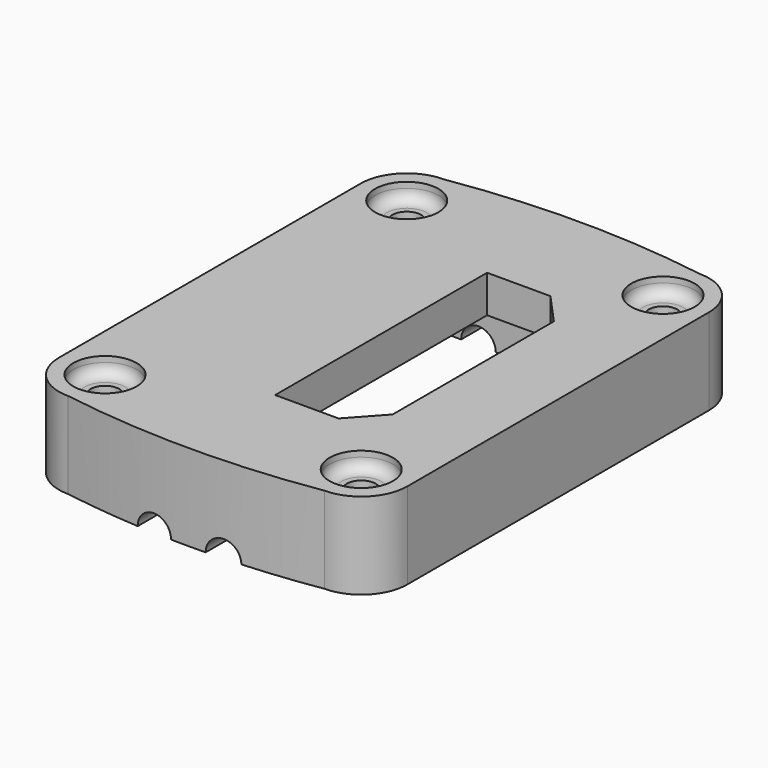
from build123d import *

# Parameters (mm, degrees)
F0_R      = 5.5
F0_R_2    = 2.5
F1_DEPTH  = 15
F2_R      = 5.5
F2_R_2    = 2.5
F3_DEPTH  = 3
F7_DEPTH  = 16
F9_DEPTH  = 8.5
F10_R     = 2
F4_R      = 3
F11_DEPTH = 43


# Not quite as in the source:
# - a feature names something its author has since deleted; it is built from what else it names


with BuildPart() as f1:
    # F0 (on Top) → F1 (new body)
    with BuildSketch(Plane.XY):
        with BuildLine():
            Line((30.2499662921, -32.75), (30.2499662921, 32.75))
            ThreePointArc((30.2499662921, 32.75), (27.9068205416, 38.4068542495), (22.2499662921, 40.75))
            ThreePointArc((22.2499662921, 40.75), (0, 42.5), (-22.2499662921, 40.75))
            ThreePointArc((-22.2499662921, 40.75), (-27.9068192027, 38.4068555884), (-30.2499662921, 32.7500037869))
            Line((-30.2499662921, 32.7500037869), (-30.2499662921, -32.75))
            ThreePointArc((-30.2499662921, -32.75), (-27.9068205416, -38.4068542495), (-22.2499662921, -40.75))
            ThreePointArc((-22.2499662921, -40.75), (0, -42.5), (22.2499662921, -40.75))
            ThreePointArc((22.2499662921, -40.75), (27.9068205416, -38.4068542495), (30.2499662921, -32.75))
        make_face()
        with Locations((-22.2499662921, -32.75)):
            Circle(F0_R, mode=Mode.SUBTRACT)
        with Locations((22.2499662921, -32.75)):
            Circle(F0_R, mode=Mode.SUBTRACT)
        with Locations((-22.2499662921, 32.75)):
            Circle(F0_R, mode=Mode.SUBTRACT)
        with Locations((22.2499662921, 32.75)):
            Circle(F0_R, mode=Mode.SUBTRACT)
        with Locations((-22.2499662921, 32.75)):
            Circle(F0_R)
        with Locations((-22.2499662921, 32.75)):
            Circle(F0_R_2, mode=Mode.SUBTRACT)
        with Locations((22.2499662921, 32.75)):
            Circle(F0_R)
        with Locations((22.2499662921, 32.75)):
            Circle(F0_R_2, mode=Mode.SUBTRACT)
        with Locations((22.2499662921, -32.75)):
            Circle(F0_R)
        with Locations((22.2499662921, -32.75)):
            Circle(F0_R_2, mode=Mode.SUBTRACT)
        with Locations((-22.2499662921, -32.75)):
            Circle(F0_R)
        with Locations((-22.2499662921, -32.75)):
            Circle(F0_R_2, mode=Mode.SUBTRACT)
    extrude(amount=F1_DEPTH)

    # F2 (on face) → F3 (cut)
    with BuildSketch(Plane.XY.offset(15)):
        with Locations((-22.2499662921, 32.75)):
            Circle(F2_R)
        with Locations((-22.2499662921, 32.75)):
            Circle(F2_R_2, mode=Mode.SUBTRACT)
        with Locations((22.2499662921, 32.75)):
            Circle(F2_R)
        with Locations((22.2499662921, 32.75)):
            Circle(F2_R_2, mode=Mode.SUBTRACT)
        with Locations((22.2499662921, -32.75)):
            Circle(F2_R)
        with Locations((22.2499662921, -32.75)):
            Circle(F2_R_2, mode=Mode.SUBTRACT)
        with Locations((-22.2499662921, -32.75)):
            Circle(F2_R)
        with Locations((-22.2499662921, -32.75)):
            Circle(F2_R_2, mode=Mode.SUBTRACT)
    extrude(amount=-F3_DEPTH, mode=Mode.SUBTRACT)

    # F6 (on Top) + F5 (on Top) → F7 (cut)
    with BuildSketch(Plane.XY):
        Polygon((-0.5, 23), (-0.5, 0), (-0.5, -23), (10.5, -23), (15.5, -17.5), (15.5, 0), (15.5, 17.5), (10.5, 23), align=None)
    with BuildSketch(Plane.XY):
        Polygon((10.5, 22.5), (0, 22.5), (0, -22.5), (10.5, -22.5), (15, -17.5), (15, 17.5), align=None)
    extrude(amount=F7_DEPTH, mode=Mode.SUBTRACT)

    # F8 (on face) → F9 (cut)
    with BuildSketch(Plane.XY):
        with BuildLine():
            Line((10.5, 23), (15.5, 17.5))
            Line((15.5, 17.5), (15.5, 25))
            ThreePointArc((15.5, 25), (14.6213203436, 27.1213203436), (12.5, 28))
            Line((12.5, 28), (-12, 28))
            ThreePointArc((-12, 28), (-14.1213203436, 27.1213203436), (-15, 25))
            Line((-15, 25), (-15, -25))
            ThreePointArc((-15, -25), (-14.1213203436, -27.1213203436), (-12, -28))
            Line((-12, -28), (12.5, -28))
            ThreePointArc((12.5, -28), (14.6213203436, -27.1213203436), (15.5, -25))
            Line((15.5, -25), (15.5, -17.5))
            Line((15.5, -17.5), (10.5, -23))
            Line((10.5, -23), (-0.5, -23))
            Line((-0.5, -23), (-0.5, 23))
            Line((-0.5, 23), (10.5, 23))
        make_face()
    extrude(amount=F9_DEPTH, mode=Mode.SUBTRACT)

    # F10
    f10_edges = [f1.edges().sort_by_distance(p)[0] for p in [
        (-27.749966, -32.75, 12),
        (16.749966, -32.75, 12),
        (-27.749966, 32.75, 12),
        (16.749966, 32.75, 12),
    ]]
    fillet(f10_edges, radius=F10_R)

    # F4 (on Front) → F11 (cut, symmetric)
    with BuildSketch(Plane.XZ):
        with Locations((6, 0)):
            Circle(F4_R)
        with Locations((-6, 0)):
            Circle(F4_R)
    extrude(amount=F11_DEPTH, both=True, mode=Mode.SUBTRACT)


solid = f1.part
